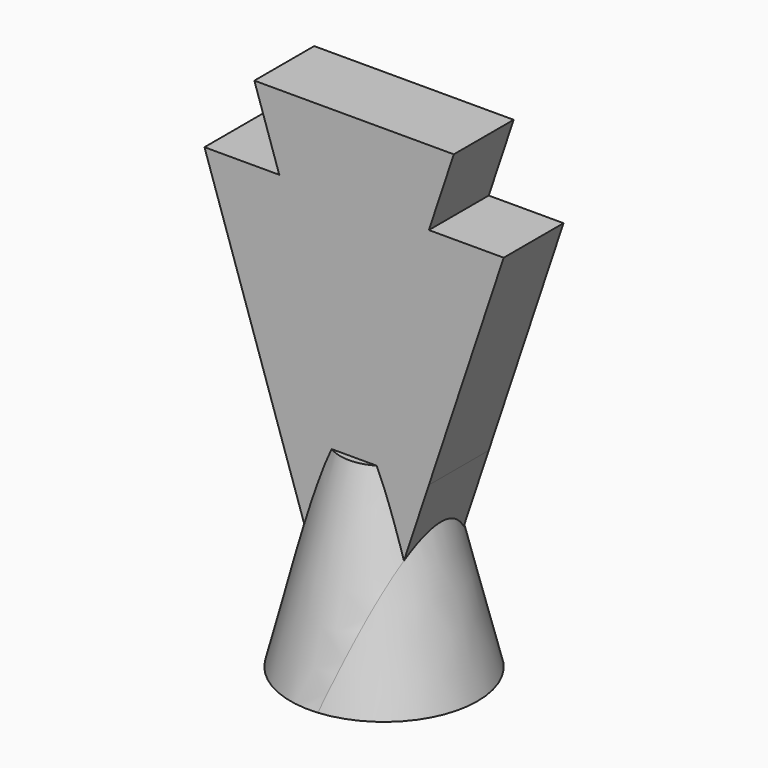
from build123d import *

# Parameters (mm, degrees)
F1_DEPTH = 15
F2_R     = 18.75
F3_DEPTH = 40


# Not quite as in the source:
# - a fillet or chamfer that OpenCascade refuses, or shapes differently, is made with other operations: its cross-section is extruded or revolved along the edge and cut away or added


with BuildPart() as f1:
    # F0 (on Front) → F1 (new body)
    with BuildSketch(Plane.XZ):
        Polygon((-15, 40.5656324383), (-35, 40.5656324383), (-30, 25.5656324383), (-15, 25.5656324383), align=None)
        Polygon((5, 40.5656324383), (-15, 40.5656324383), (-15, 25.5656324383), (0, 25.5656324383), align=None)
        Polygon((-15, 25.5656324383), (-30, 25.5656324383), (-45, 25.5656324383), (-30, -19.4343675617), (0, -19.4343675617), (15, 25.5656324383), (0, 25.5656324383), align=None)
    extrude(amount=F1_DEPTH)

    # F2 (on face) → F3 (join)
    with BuildSketch(Plane(origin=(0, 0, -19.4343675617), x_dir=(1, 0, 0), z_dir=(0, 0, -1))):
        with Locations((-15, 7.5)):
            Circle(F2_R)
    extrude(amount=F3_DEPTH)

    # F4: chamfer of 10 x 40 on 1 edges, made by hand


with BuildPart() as f4_tool2:
    # F4_s3 → F4_t4 (revolve)
    with BuildSketch(Plane.XZ.offset(7.5)):
        Polygon((3.75, -59.4343675617), (-6.25, -19.4343675617), (3.75, -19.4343675617), align=None)
    revolve(axis=Axis((-15, -7.5, -19.4343675617), (0, 0, -1)))

    split(bisect_by=Plane(origin=(5.8303102685, 0, -1.9434367562), x_dir=(0, 1, 0), z_dir=(0.9486832981, 0, -0.316227766)), keep=Keep.TOP)


with BuildPart() as f1_1:
    add(f1.part)

    # F4_t1: cut F4_tool2
    add(f4_tool2.part, mode=Mode.SUBTRACT)


with BuildPart() as f4_tool7:
    # F4_s8 → F4_t9 (revolve)
    with BuildSketch(Plane.XZ.offset(7.5)):
        Polygon((3.75, -59.4343675617), (-6.25, -19.4343675617), (3.75, -19.4343675617), align=None)
    revolve(axis=Axis((-15, -7.5, -19.4343675617), (0, 0, -1)))

    split(bisect_by=Plane.XZ.offset(15), keep=Keep.TOP)


with BuildPart() as f1_2:
    add(f1_1.part)

    # F4_t6: cut F4_tool7
    add(f4_tool7.part, mode=Mode.SUBTRACT)


with BuildPart() as f4_tool12:
    # F4_s13 → F4_t14 (revolve)
    with BuildSketch(Plane.XZ.offset(7.5)):
        Polygon((3.75, -59.4343675617), (-6.25, -19.4343675617), (3.75, -19.4343675617), align=None)
    revolve(axis=Axis((-15, -7.5, -19.4343675617), (0, 0, -1)))

    split(bisect_by=Plane.XZ, keep=Keep.BOTTOM)


with BuildPart() as f1_3:
    add(f1_2.part)

    # F4_t11: cut F4_tool12
    add(f4_tool12.part, mode=Mode.SUBTRACT)


with BuildPart() as f4_tool17:
    # F4_s18 → F4_t19 (revolve)
    with BuildSketch(Plane.XZ.offset(7.5)):
        Polygon((3.75, -59.4343675617), (-6.25, -19.4343675617), (3.75, -19.4343675617), align=None)
    revolve(axis=Axis((-15, -7.5, -19.4343675617), (0, 0, -1)))

    split(bisect_by=Plane(origin=(-32.8303102685, 0, -10.9434367562), x_dir=(0, 1, 0), z_dir=(-0.9486832981, 0, -0.316227766)), keep=Keep.TOP)


with BuildPart() as f1_4:
    add(f1_3.part)

    # F4_t16: cut F4_tool17
    add(f4_tool17.part, mode=Mode.SUBTRACT)


solid = f1_4.part
